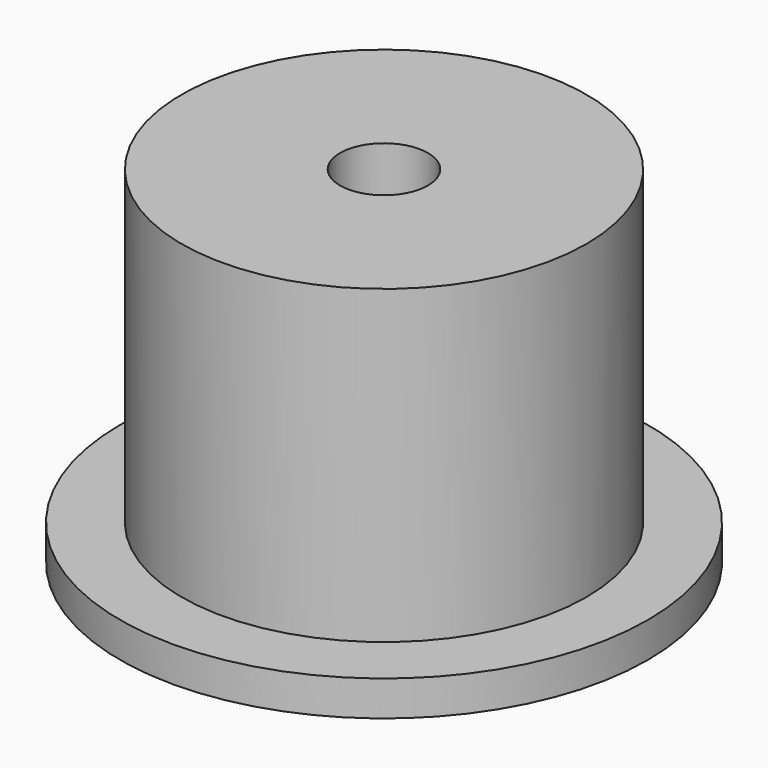
from build123d import *

# Parameters (mm, degrees)
F0_R     = 17.25
F0_R_2   = 3.75
F1_DEPTH = 26.5
F2_R     = 22.5
F2_R_2   = 17.25
F2_R_3   = 3.75
F3_DEPTH = 3


with BuildPart() as f1:
    # F0 (on Top) → F1 (new body)
    with BuildSketch(Plane.XY):
        Circle(F0_R)
        Circle(F0_R_2, mode=Mode.SUBTRACT)
    extrude(amount=F1_DEPTH)

    # F2 (on face) → F3 (join)
    with BuildSketch(Plane(origin=(0, 0, 0), x_dir=(1, 0, 0), z_dir=(0, 0, -1))):
        Circle(F2_R)
        Circle(F2_R_2, mode=Mode.SUBTRACT)
        Circle(F2_R_2)
        Circle(F2_R_3, mode=Mode.SUBTRACT)
    extrude(amount=F3_DEPTH)


solid = f1.part
